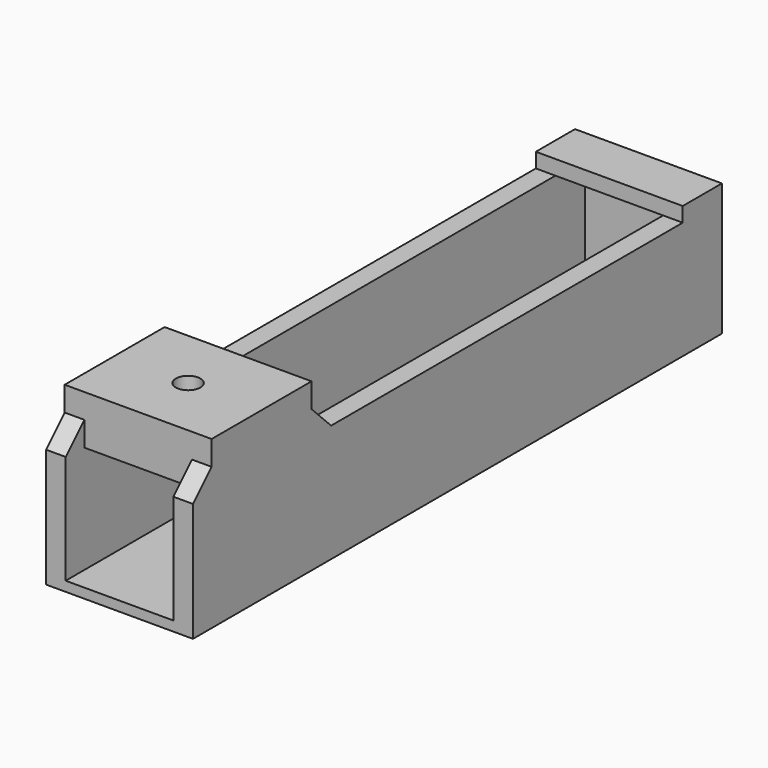
from build123d import *

# Parameters (mm, degrees)
F1_DEPTH     = 22
F2_W         = 30
F2_H         = 135
F3_DEPTH     = 2
F4_W         = 30
F4_H         = 25.5063175828
F4_R         = 2.5
F5_DEPTH     = 10
F6_W         = 30
F6_H         = 10
F7_DEPTH     = 3
F8_T1_DEPTH  = 4
F8_T3_DEPTH  = 4
F8_T8_DEPTH  = 4
F8_T13_DEPTH = 4


# Not quite as in the source:
# - a fillet or chamfer that OpenCascade refuses, or shapes differently, is made with other operations: its cross-section is extruded or revolved along the edge and cut away or added


with BuildPart() as f1:
    # F0 (on Top) → F1 (new body)
    with BuildSketch(Plane.XY):
        Polygon((160.7300297916, 27.1383413836), (130.7300297916, 27.1383413836), (130.7300297916, -107.8616586164), (134.7300297916, -107.8616586164), (134.7300297916, -105.3616586164), (134.7300297916, 24.6383413836), (156.7300297916, 24.6383413836), (156.7300297916, -105.3616586164), (156.7300297916, -107.8616586164), (160.7300297916, -107.8616586164), align=None)
    extrude(amount=F1_DEPTH)

    # F2 (on face) → F3 (join)
    with BuildSketch(Plane(origin=(0, 0, 0), x_dir=(1, 0, 0), z_dir=(0, 0, -1))):
        with Locations((145.7300297916, 40.3616586164)):
            Rectangle(F2_W, F2_H)
    extrude(amount=F3_DEPTH)

    # F4 (on face) → F5 (join)
    with BuildSketch(Plane.XY.offset(22)):
        with Locations((145.7300297916, -90.3616586164)):
            Rectangle(F4_W, F4_H)
        with Locations((145.7300297916, -90.3616586164)):
            Circle(F4_R, mode=Mode.SUBTRACT)
    extrude(amount=F5_DEPTH)

    # F6 (on face) → F7 (join)
    with BuildSketch(Plane.XY.offset(22)):
        with Locations((145.7300297916, 22.1383413836)):
            Rectangle(F6_W, F6_H)
    extrude(amount=F7_DEPTH)

    # F8: chamfer of 5 on 4 edges, made by hand

    # F8_s2 → F8_t1 (join)
    with BuildSketch(Plane.YZ.offset(156.7300297916)):
        Polygon((-72.608499825, 22), (-77.608499825, 27), (-77.608499825, 22), align=None)
    extrude(amount=F8_T1_DEPTH)

    # F8_s4 → F8_t3 (join)
    with BuildSketch(Plane.YZ.offset(130.7300297916)):
        Polygon((-77.608499825, 27), (-72.608499825, 22), (-77.608499825, 22), align=None)
    extrude(amount=F8_T3_DEPTH)


with BuildPart() as f8_tool6:
    # F8_s7 → F8_t8 (new body)
    with BuildSketch(Plane.YZ.offset(130.7300297916)):
        Polygon((-103.1148174078, 27), (-108.1148174078, 22), (-103.1148174078, 22), align=None)
    extrude(amount=F8_T8_DEPTH)

    split(bisect_by=Plane.XZ.offset(107.8616586164), keep=Keep.BOTTOM)


with BuildPart() as f1_1:
    add(f1.part)

    # F8_t5: union F8_tool6
    add(f8_tool6.part)


with BuildPart() as f8_tool11:
    # F8_s12 → F8_t13 (new body)
    with BuildSketch(Plane.YZ.offset(156.7300297916)):
        Polygon((-103.1148174078, 27), (-108.1148174078, 22), (-103.1148174078, 22), align=None)
    extrude(amount=F8_T13_DEPTH)

    split(bisect_by=Plane.XZ.offset(107.8616586164), keep=Keep.BOTTOM)


with BuildPart() as f1_2:
    add(f1_1.part)

    # F8_t10: union F8_tool11
    add(f8_tool11.part)


solid = f1_2.part
